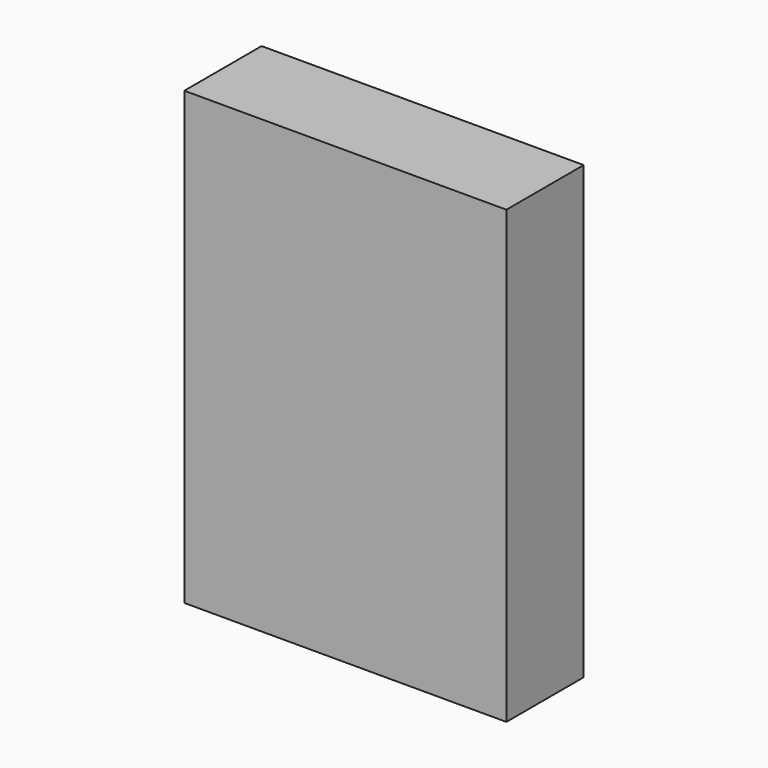
from build123d import *

# Parameters (mm, degrees)
F0_W     = 63.5
F0_H     = 88.9
F1_DEPTH = 19.05


# Not quite as in the source:
# - a length typed as a fraction of an inch, garbled in the dataset ("3 / 203.2 mm" for 3/8 in), is restored


with BuildPart() as f1:
    # F0 (on Front) → F1 (new body)
    with BuildSketch(Plane.XZ):
        with Locations((31.75, 44.45)):
            Rectangle(F0_W, F0_H)
    extrude(amount=F1_DEPTH)


solid = f1.part
